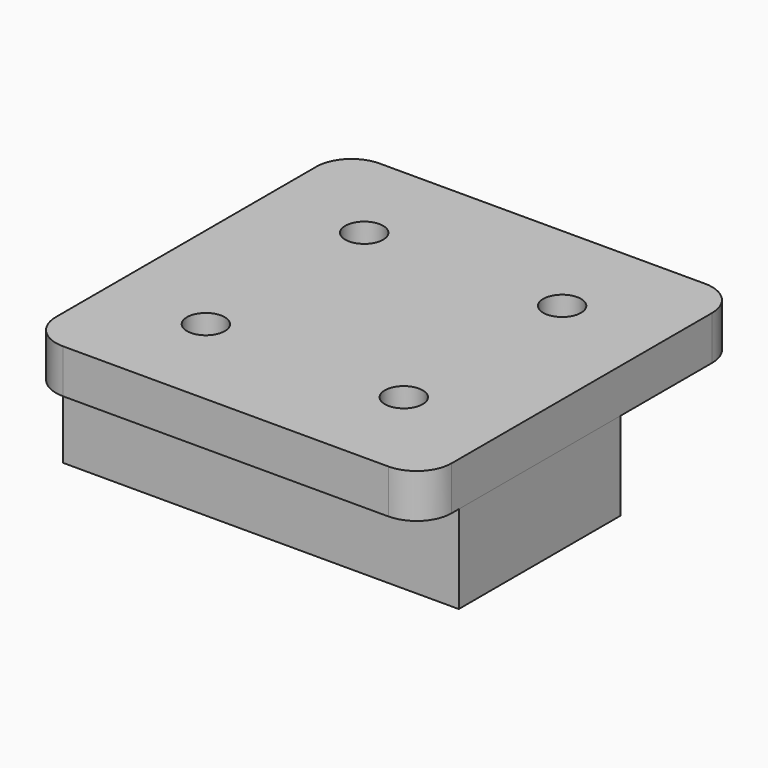
from build123d import *

# Parameters (mm, degrees)
F0_R     = 2.15
F2_DEPTH = 5
F1_W     = 45
F1_H     = 23
F1_R     = 4
F1_R_2   = 2.15
F3_DEPTH = 10
F4_DEPTH = 3.5
F5_DEPTH = 2
F6_DEPTH = 10
F7_R     = 4
F7_R_2   = 2.15
F8_DEPTH = 5


# Not quite as in the source:
# - a feature names something its author has since deleted; it is built from what else it names


with BuildPart() as f2:
    # F0 (on Top) → F2 (new body)
    with BuildSketch(Plane.XY):
        with BuildLine():
            ThreePointArc((5, -1), (6.1715728753, -3.8284271247), (9, -5))
            Line((9, -5), (46, -5))
            ThreePointArc((46, -5), (48.8284271247, -3.8284271247), (50, -1))
            Line((50, -1), (50, 36))
            ThreePointArc((50, 36), (48.8284271247, 38.8284271247), (46, 40))
            Line((46, 40), (9, 40))
            ThreePointArc((9, 40), (6.1715728753, 38.8284271247), (5, 36))
            Line((5, 36), (5, -1))
        make_face()
        with Locations((16.25, 6.25)):
            Circle(F0_R, mode=Mode.SUBTRACT)
        with Locations((38.75, 6.25)):
            Circle(F0_R, mode=Mode.SUBTRACT)
        with Locations((16.25, 28.75)):
            Circle(F0_R, mode=Mode.SUBTRACT)
        with Locations((38.75, 28.75)):
            Circle(F0_R, mode=Mode.SUBTRACT)
        with Locations((16.25, 6.25)):
            Circle(F0_R)
        with Locations((38.75, 6.25)):
            Circle(F0_R)
    extrude(amount=F2_DEPTH)

    # F1 (on Top) → F5 (cut)
    with BuildSketch(Plane.XY):
        with Locations((34.35, 18)):
            Circle(F1_R_2)
        with Locations((20.65, 18)):
            Circle(F1_R_2)
    extrude(amount=F5_DEPTH, mode=Mode.SUBTRACT)


with BuildPart() as f3:
    # F1 (on Top) → F3 (new body)
    with BuildSketch(Plane.XY):
        with Locations((27.5, 11.5)):
            Rectangle(F1_W, F1_H)
        with Locations((12, 18)):
            Circle(F1_R, mode=Mode.SUBTRACT)
        Polygon((20.65, 22.3301270189), (24.4, 20.1650635095), (24.4, 15.8349364905), (20.65, 13.6698729811), (16.9, 15.8349364905), (16.9, 20.1650635095), align=None, mode=Mode.SUBTRACT)
        Polygon((34.35, 13.6698729811), (30.6, 15.8349364905), (30.6, 20.1650635095), (34.35, 22.3301270189), (38.1, 20.1650635095), (38.1, 15.8349364905), align=None, mode=Mode.SUBTRACT)
        with Locations((43, 18)):
            Circle(F1_R, mode=Mode.SUBTRACT)
        Polygon((24.4, 15.8349364905), (24.4, 20.1650635095), (20.65, 22.3301270189), (16.9, 20.1650635095), (16.9, 15.8349364905), (20.65, 13.6698729811), align=None)
        with Locations((20.65, 18)):
            Circle(F1_R_2, mode=Mode.SUBTRACT)
        Polygon((30.6, 20.1650635095), (30.6, 15.8349364905), (34.35, 13.6698729811), (38.1, 15.8349364905), (38.1, 20.1650635095), (34.35, 22.3301270189), align=None)
        with Locations((34.35, 18)):
            Circle(F1_R_2, mode=Mode.SUBTRACT)
    extrude(amount=-F3_DEPTH)

    # F1 (on Top) → F4 (cut)
    with BuildSketch(Plane.XY):
        Polygon((24.4, 15.8349364905), (24.4, 20.1650635095), (20.65, 22.3301270189), (16.9, 20.1650635095), (16.9, 15.8349364905), (20.65, 13.6698729811), align=None)
        with Locations((20.65, 18)):
            Circle(F1_R_2, mode=Mode.SUBTRACT)
        Polygon((30.6, 20.1650635095), (30.6, 15.8349364905), (34.35, 13.6698729811), (38.1, 15.8349364905), (38.1, 20.1650635095), (34.35, 22.3301270189), align=None)
        with Locations((34.35, 18)):
            Circle(F1_R_2, mode=Mode.SUBTRACT)
    extrude(amount=-F4_DEPTH, mode=Mode.SUBTRACT)


with BuildPart() as f6_tool:
    # F0 (on Top) → F6 (new body, symmetric)
    with BuildSketch(Plane.XY):
        with Locations((16.25, 6.25)):
            Circle(F0_R)
        with Locations((38.75, 6.25)):
            Circle(F0_R)
    extrude(amount=F6_DEPTH, both=True)


with BuildPart() as f2_1:
    add(f2.part)

    # F6: cut by f6_tool
    add(f6_tool.part, mode=Mode.SUBTRACT)


with BuildPart() as f3_1:
    add(f3.part)

    # F6: cut by f6_tool
    add(f6_tool.part, mode=Mode.SUBTRACT)

    # F7 (on face) → F8 (cut)
    with BuildSketch(Plane(origin=(0, 0, -10), x_dir=(1, 0, 0), z_dir=(0, 0, -1))):
        with Locations((16.25, -6.25)):
            Circle(F7_R)
        with Locations((16.25, -6.25)):
            Circle(F7_R_2, mode=Mode.SUBTRACT)
        with Locations((38.75, -6.25)):
            Circle(F7_R)
        with Locations((38.75, -6.25)):
            Circle(F7_R_2, mode=Mode.SUBTRACT)
    extrude(amount=-F8_DEPTH, mode=Mode.SUBTRACT)


solid = Compound([f2_1.part, f3_1.part])
